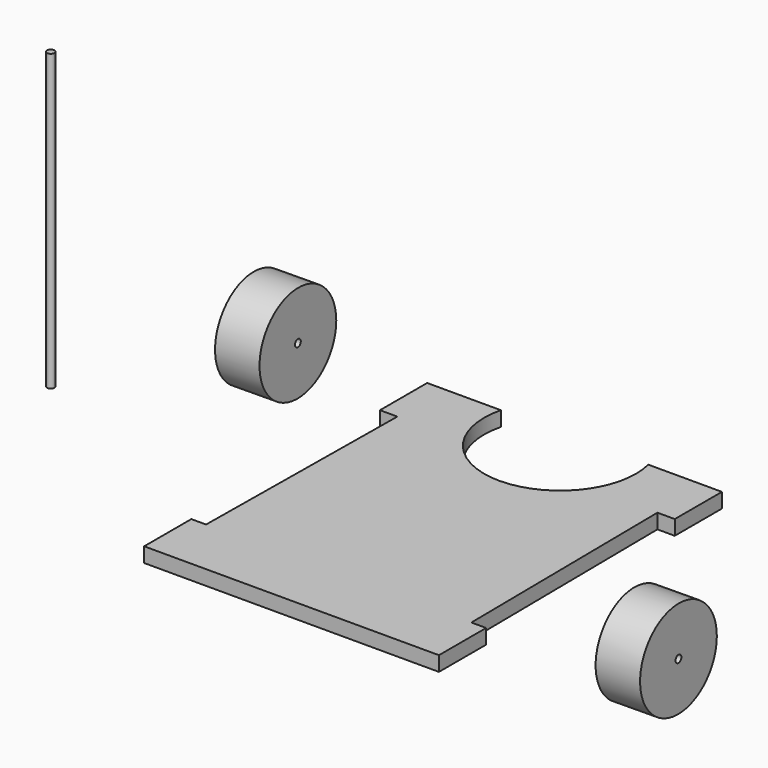
from build123d import *

# Parameters (mm, degrees)
F0_W     = 22.86
F0_H     = 31.75
F0_W_2   = 24.13
F0_H_2   = 25.4
F1_DEPTH = 6.35
F2_R     = 20.955
F2_R_2   = 1.5875
F3_DEPTH = 19
F4_DEPTH = 18.9992
F5_R     = 1.5875
F6_DEPTH = 127


with BuildPart() as f1:
    # F0 (on Top) → F1 (new body)
    with BuildSketch(Plane.XY):
        with BuildLine():
            Line((72.7303429186, 98.2907311208), (40.9803429186, 98.2907311208))
            ThreePointArc((40.9803429186, 98.2907311208), (40.5288228565, 81.0386007186), (31.3563980824, 66.4198970297))
            Line((31.3563980824, 66.4198970297), (33.3603429186, 66.4198970297))
            Line((33.3603429186, 66.4198970297), (33.3603429186, -9.7801029703))
            Line((33.3603429186, -9.7801029703), (9.2303429186, -9.7801029703))
            Line((9.2303429186, -9.7801029703), (9.2303429186, -16.1301029703))
            Line((9.2303429186, -16.1301029703), (33.3603429186, -16.1301029703))
            Line((33.3603429186, -16.1301029703), (33.3603429186, -41.5301029703))
            Line((33.3603429186, -41.5301029703), (9.2303429186, -41.5301029703))
            Line((9.2303429186, -41.5301029703), (9.2303429186, -54.1092688792))
            Line((9.2303429186, -54.1092688792), (72.7303429186, -54.1092688792))
            Line((72.7303429186, -54.1092688792), (72.7303429186, -28.7092688792))
            Line((72.7303429186, -28.7092688792), (66.3803429186, -28.7092688792))
            Line((66.3803429186, -28.7092688792), (65.2497625203, 72.8907311208))
            Line((65.2497625203, 72.8907311208), (72.7303429186, 72.8907311208))
            Line((72.7303429186, 72.8907311208), (72.7303429186, 98.2907311208))
        make_face()
        with Locations((47.9653429186, 12.4448970297)):
            Rectangle(F0_W, F0_H, mode=Mode.SUBTRACT)
        with BuildLine():
            Line((-22.5196570814, 98.2907311208), (-54.2696570814, 98.2907311208))
            Line((-54.2696570814, 98.2907311208), (-54.2696570814, 72.8907311208))
            Line((-54.2696570814, 72.8907311208), (-46.789076683, 72.8907311208))
            Line((-46.789076683, 72.8907311208), (-47.9196570814, -28.7092688792))
            Line((-47.9196570814, -28.7092688792), (-54.2696570814, -28.7092688792))
            Line((-54.2696570814, -28.7092688792), (-54.2696570814, -54.1092688792))
            Line((-54.2696570814, -54.1092688792), (9.2303429186, -54.1092688792))
            Line((9.2303429186, -54.1092688792), (9.2303429186, -41.5301029703))
            Line((9.2303429186, -41.5301029703), (-14.8996570814, -41.5301029703))
            Line((-14.8996570814, -41.5301029703), (-14.8996570814, -16.1301029703))
            Line((-14.8996570814, -16.1301029703), (9.2303429186, -16.1301029703))
            Line((9.2303429186, -16.1301029703), (9.2303429186, -9.7801029703))
            Line((9.2303429186, -9.7801029703), (-14.8996570814, -9.7801029703))
            Line((-14.8996570814, -9.7801029703), (-14.8996570814, 66.4198970297))
            Line((-14.8996570814, 66.4198970297), (-12.8957122452, 66.4198970297))
            ThreePointArc((-12.8957122452, 66.4198970297), (-22.0681370192, 81.0386007186), (-22.5196570814, 98.2907311208))
        make_face()
        with Locations((-29.5046570814, 12.4448970297)):
            Rectangle(F0_W, F0_H, mode=Mode.SUBTRACT)
        with Locations((-2.8346570814, -28.8301029703)):
            Rectangle(F0_W_2, F0_H_2)
        with Locations((21.2953429186, -28.8301029703)):
            Rectangle(F0_W_2, F0_H_2)
        with BuildLine():
            ThreePointArc((31.3563980824, 66.4198970297), (21.1040989763, 60.027732272), (9.2303429186, 57.7953962005))
            Line((9.2303429186, 57.7953962005), (9.2303429186, -9.7801029703))
            Line((9.2303429186, -9.7801029703), (33.3603429186, -9.7801029703))
            Line((33.3603429186, -9.7801029703), (33.3603429186, 66.4198970297))
            Line((33.3603429186, 66.4198970297), (31.3563980824, 66.4198970297))
        make_face()
        with BuildLine():
            ThreePointArc((9.2303429186, 57.7953962005), (-2.643413139, 60.027732272), (-12.8957122452, 66.4198970297))
            Line((-12.8957122452, 66.4198970297), (-14.8996570814, 66.4198970297))
            Line((-14.8996570814, 66.4198970297), (-14.8996570814, -9.7801029703))
            Line((-14.8996570814, -9.7801029703), (9.2303429186, -9.7801029703))
            Line((9.2303429186, -9.7801029703), (9.2303429186, 57.7953962005))
        make_face()
        with Locations((-29.5046570814, 12.4448970297)):
            Rectangle(F0_W, F0_H)
        with Locations((47.9653429186, 12.4448970297)):
            Rectangle(F0_W, F0_H)
    extrude(amount=F1_DEPTH)


with BuildPart() as f3:
    # F2 (on face) → F3 (new body)
    with BuildSketch(Plane(origin=(66.0526939603, 0.7350185143, 0), x_dir=(-0.0111270709, 0.9999380922, 0), z_dir=(0.9999380922, 0.0111270709, 0))):
        with Locations((-148.4907998811, 167.2162994118)):
            Circle(F2_R)
        with Locations((-148.4907998811, 167.2162994118)):
            Circle(F2_R_2, mode=Mode.SUBTRACT)
    extrude(amount=F3_DEPTH)


with BuildPart() as f4:
    # F2 (on face) → F4 (new body)
    with BuildSketch(Plane(origin=(66.0526939603, 0.7350185143, 0), x_dir=(-0.0111270709, 0.9999380922, 0), z_dir=(0.9999380922, 0.0111270709, 0))):
        with Locations((59.3689817467, -37.7408552219)):
            Circle(F2_R)
        with Locations((59.3689817467, -37.7408552219)):
            Circle(F2_R_2, mode=Mode.SUBTRACT)
    extrude(amount=F4_DEPTH)


with BuildPart() as f4b:
    # F2 (on face) → F4, piece 2 (new body)
    with BuildSketch(Plane(origin=(66.0526939603, 0.7350185143, 0), x_dir=(-0.0111270709, 0.9999380922, 0), z_dir=(0.9999380922, 0.0111270709, 0))):
        with Locations((-148.4907998811, 167.2162994118)):
            Circle(F2_R)
        with Locations((-148.4907998811, 167.2162994118)):
            Circle(F2_R_2, mode=Mode.SUBTRACT)
    extrude(amount=F4_DEPTH)


with BuildPart() as f6:
    # F5 (on Top) → F6 (new body)
    with BuildSketch(Plane.XY):
        with Locations((-159.145578742, 26.7000477761)):
            Circle(F5_R)
    extrude(amount=F6_DEPTH)


solid = Compound([f1.part, f3.part, f4.part, f4b.part, f6.part])
